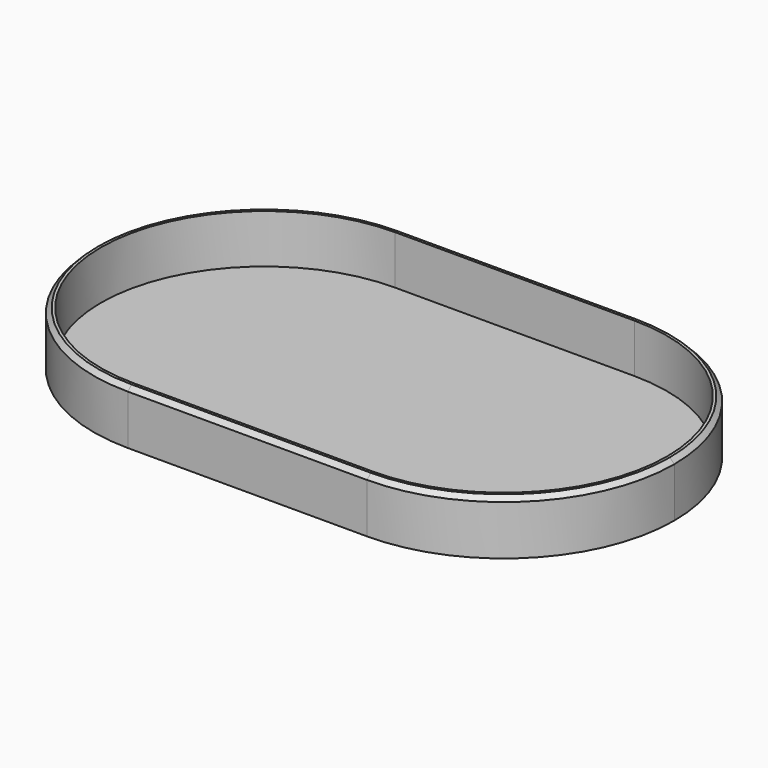
from build123d import *

# Parameters (mm, degrees)
F1_DEPTH = 6
F3_DEPTH = 5.4
F4_SIZE  = 0.5


with BuildPart() as f1:
    # F0 (on Top) → F1 (new body)
    with BuildSketch(Plane.XY):
        with BuildLine():
            Line((13.25, 18.9), (-13.25, 18.9))
            ThreePointArc((-13.25, 18.9), (-26.6143181644, 13.3643181644), (-32.15, 0))
            ThreePointArc((-32.15, 0), (-26.6143181644, -13.3643181644), (-13.25, -18.9))
            Line((-13.25, -18.9), (13.25, -18.9))
            ThreePointArc((13.25, -18.9), (26.6143181644, -13.3643181644), (32.15, 0))
            ThreePointArc((32.15, 0), (26.6143181644, 13.3643181644), (13.25, 18.9))
        make_face()
    extrude(amount=F1_DEPTH)

    # F2 (on face) → F3 (cut)
    with BuildSketch(Plane.XY.offset(6)):
        with BuildLine():
            Line((13.25, 18.1), (-13.25, 18.1))
            ThreePointArc((-13.25, 18.1), (-31.35, 0), (-13.25, -18.1))
            Line((-13.25, -18.1), (13.25, -18.1))
            ThreePointArc((13.25, -18.1), (31.35, 0), (13.25, 18.1))
        make_face()
    extrude(amount=-F3_DEPTH, mode=Mode.SUBTRACT)

    # F4
    f4_edges = [f1.edges().sort_by_distance(p)[0] for p in [
        (-32.15, 0, 6),
        (32.15, 0, 6),
        (0, 18.9, 6),
        (0, -18.9, 6),
    ]]
    chamfer(f4_edges, length=F4_SIZE)


solid = f1.part
